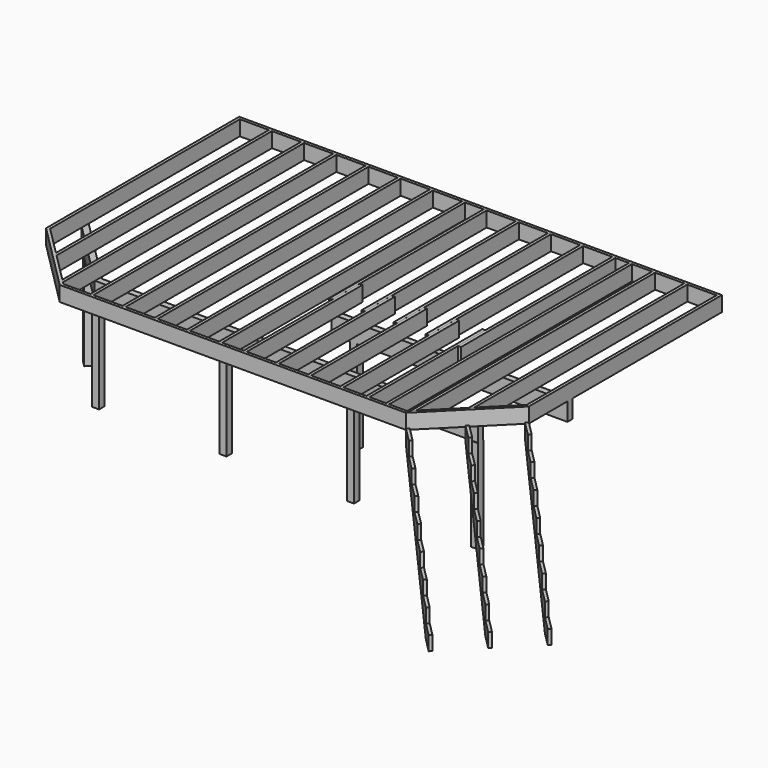
from build123d import *

# Parameters (mm, degrees)
F2_DEPTH       = 190.246
F3_W           = 38.1
F3_H           = 3833.9045876226
F3_H_2         = 2438.4
F4_DEPTH       = 190.754
F5_W           = 38.1
F5_H           = 3833.9045876226
F5_H_2         = 1828.8
F6_DEPTH       = 190.5
F7_W           = 2978.15
F7_H           = 76.2
F8_DEPTH       = 228.6
F13_DEPTH      = 38.1
F15_DEPTH      = 19.05
F15_DEPTH_BACK = 19.05
F17_DEPTH      = 38.1
F19_W          = 88.9
F19_H          = 88.9
F20_DEPTH      = 1180.846


with BuildPart() as f2:
    # F1 (on Top) → F2 (new body)
    with BuildSketch(Plane.XY):
        Polygon((0, -38.1), (0, 0), (-2971.8, 0), (-2971.8, -38.1), (-38.1, -38.1), align=None)
        Polygon((-2971.8, -38.1), (-2971.8, 0), (-6096, 0), (-6096, -38.1), (-6057.9, -38.1), align=None)
        Polygon((0, -3048), (0, -38.1), (-38.1, -38.1), (-38.1, -3032.2184632736), align=None)
        Polygon((-862.1045876226, -3910.1045876226), (0, -3048), (-38.1, -3032.2184632736), (-877.8861243491, -3872.0045876226), (-5218.1138756509, -3872.0045876226), (-5233.8954123774, -3910.1045876226), align=None)
        Polygon((-6057.9, -3032.2184632736), (-6057.9, -38.1), (-6096, -38.1), (-6096, -3048), align=None)
        Polygon((-5218.1138756509, -3872.0045876226), (-6057.9, -3032.2184632736), (-6096, -3048), (-5233.8954123774, -3910.1045876226), align=None)
    extrude(amount=F2_DEPTH)

    # F3 (on Top) → F4 (join)
    with BuildSketch(Plane.XY):
        Polygon((-406.4, -3400.5184632736), (-406.4, -34.379438989), (-444.5, -37.4872828711), (-444.5, -3438.6184632736), align=None)
        Polygon((-812.8, -38.1), (-850.9, -38.1), (-850.9, -3845.0184632736), (-812.8, -3806.9184632736), align=None)
        with Locations((-1123.95, -1955.0522938113)):
            Rectangle(F3_W, F3_H)
        with Locations((-1333.5, -1257.3)):
            Rectangle(F3_W, F3_H_2)
        with Locations((-1739.9, -1257.3)):
            Rectangle(F3_W, F3_H_2)
        with Locations((-2146.3, -1257.3)):
            Rectangle(F3_W, F3_H_2)
        with Locations((-2552.7, -1257.3)):
            Rectangle(F3_W, F3_H_2)
        with Locations((-2959.1, -1257.3)):
            Rectangle(F3_W, F3_H_2)
    extrude(amount=F4_DEPTH)

    # F5 (on Top) → F6 (join)
    with BuildSketch(Plane.XY):
        Polygon((-5651.5, -38.1), (-5689.6, -38.1), (-5689.6, -3400.5184632736), (-5651.5, -3438.6184632736), align=None)
        Polygon((-5245.1, -38.1), (-5283.2, -38.1), (-5283.2, -3806.9184632736), (-5245.1, -3845.0184632736), align=None)
        with Locations((-4857.75, -1955.0522938113)):
            Rectangle(F5_W, F5_H)
        with Locations((-4451.35, -1955.0522938113)):
            Rectangle(F5_W, F5_H)
        with Locations((-4044.95, -1955.0522938113)):
            Rectangle(F5_W, F5_H)
        with Locations((-3638.55, -1955.0522938113)):
            Rectangle(F5_W, F5_H)
        with Locations((-3232.15, -1955.0522938113)):
            Rectangle(F5_W, F5_H)
        with Locations((-2921, -2957.6045876226)):
            Rectangle(F5_W, F5_H_2)
        with Locations((-2514.6, -2957.6045876226)):
            Rectangle(F5_W, F5_H_2)
        with Locations((-2108.2, -2957.6045876226)):
            Rectangle(F5_W, F5_H_2)
        with Locations((-1701.8, -2957.6045876226)):
            Rectangle(F5_W, F5_H_2)
        with Locations((-1371.6, -2957.6045876226)):
            Rectangle(F5_W, F5_H_2)
    extrude(amount=F6_DEPTH)

    # F7 (on Top) → F8 (join)
    with BuildSketch(Plane.XY):
        with Locations((-1489.075, -2400.3)):
            Rectangle(F7_W, F7_H)
        Polygon((-406.4, -3338.6045876226), (-406.4, -3262.4045876226), (-5218.1138756509, -3262.4045876226), (-5249.6769491038, -3338.6045876226), align=None)
        Polygon((-5249.6769491038, -3338.6045876226), (-5218.1138756509, -3262.4045876226), (-6096, -2384.5184632736), (-6096, -2492.2815367264), align=None)
    extrude(amount=-F8_DEPTH)

    # F12 (on face) → F13 (join)
    with BuildSketch(Plane(origin=(-1524, -1524, 0), x_dir=(0.7071067812, -0.7071067812, 0), z_dir=(-0.7071067812, -0.7071067812, 0))):
        Polygon((2409.2614690566, 12.954), (2155.2614690566, 12.954), (2155.2614690566, -165.7994895356), (3931.8993411486, -1409.446), (4187.2614690566, -1409.446), (4187.2614690566, -1231.646), (3933.2614690566, -1231.646), (3933.2614690566, -1053.846), (3679.2614690566, -1053.846), (3679.2614690566, -876.046), (3425.2614690566, -876.046), (3425.2614690566, -698.246), (3171.2614690566, -698.246), (3171.2614690566, -520.446), (2917.2614690566, -520.446), (2917.2614690566, -342.646), (2663.2614690566, -342.646), (2663.2614690566, -164.846), (2409.2614690566, -164.846), align=None)
    extrude(amount=F13_DEPTH)

    # F14 (on face) → F15 (join, two sides)
    with BuildSketch(Plane(origin=(-1955.0522938113, -1955.0522938113, 0), x_dir=(0.7071067812, -0.7071067812, 0), z_dir=(-0.7071067812, -0.7071067812, 0))) as f15_sk:
        Polygon((2409.2614690566, 12.954), (2155.2614690566, 12.954), (2155.2614690566, -165.7994895356), (3931.8993411486, -1409.446), (4187.2614690566, -1409.446), (4187.2614690566, -1231.646), (3933.2614690566, -1231.646), (3933.2614690566, -1053.846), (3679.2614690566, -1053.846), (3679.2614690566, -876.046), (3425.2614690566, -876.046), (3425.2614690566, -698.246), (3171.2614690566, -698.246), (3171.2614690566, -520.446), (2917.2614690566, -520.446), (2917.2614690566, -342.646), (2663.2614690566, -342.646), (2663.2614690566, -164.846), (2409.2614690566, -164.846), align=None)
    extrude(amount=F15_DEPTH)
    extrude(f15_sk.sketch, amount=-F15_DEPTH_BACK)

    # F16 (on face) → F17 (join)
    with BuildSketch(Plane(origin=(-2386.1045876226, -2386.1045876226, 0), x_dir=(0.7071067812, -0.7071067812, 0), z_dir=(-0.7071067812, -0.7071067812, 0))):
        Polygon((2409.2614690566, 12.954), (2155.2614690566, 12.954), (2155.2614690566, -165.7994895356), (3931.8993411486, -1409.446), (4187.2614690566, -1409.446), (4187.2614690566, -1231.646), (3933.2614690566, -1231.646), (3933.2614690566, -1053.846), (3679.2614690566, -1053.846), (3679.2614690566, -876.046), (3425.2614690566, -876.046), (3425.2614690566, -698.246), (3171.2614690566, -698.246), (3171.2614690566, -520.446), (2917.2614690566, -520.446), (2917.2614690566, -342.646), (2663.2614690566, -342.646), (2663.2614690566, -164.846), (2409.2614690566, -164.846), align=None)
    extrude(amount=-F17_DEPTH)

    # F19 (on offset) → F20 (join, through all)
    with BuildSketch(Plane.XY.offset(-228.6)):
        with Locations((-2698.75, -2393.95)):
            Rectangle(F19_W, F19_H)
        Polygon((-5817.6120602469, -2653.9261469057), (-5880.4738530943, -2591.0643540582), (-5943.3356459418, -2653.9261469057), (-5880.4738530943, -2716.7879397531), align=None)
        with Locations((-5233.8954123774, -3300.5045876226)):
            Rectangle(F19_W, F19_H)
        with Locations((-450.85, -3300.5045876226)):
            Rectangle(F19_W, F19_H)
        with Locations((-2015.5651374591, -3300.5045876226)):
            Rectangle(F19_W, F19_H)
        with Locations((-3624.7302749182, -3300.5045876226)):
            Rectangle(F19_W, F19_H)
    extrude(amount=-F20_DEPTH)


solid = f2.part
